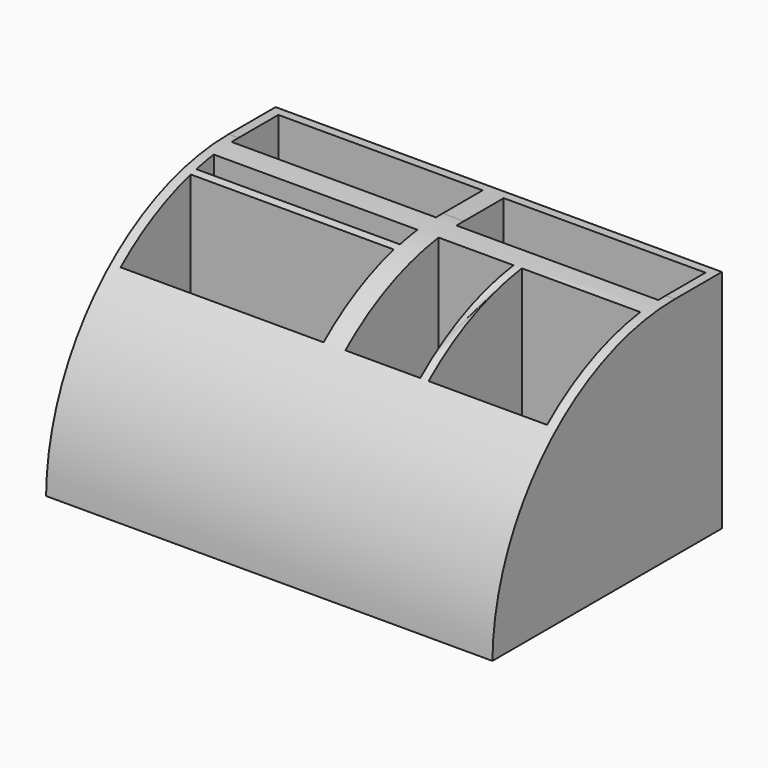
from build123d import *

# Parameters (mm, degrees)
F0_W        = 198.8127231598
F0_H        = 127.7878135443
F1_DEPTH    = 100.584
F2_T1_DEPTH = 706.7873225248
F3_W        = 90.9917657264
F3_H        = 25.9568989277
F4_DEPTH    = 88.392
F5_W        = 89.8508075625
F5_H        = 26.2421388179
F6_DEPTH    = 88.646
F7_DEPTH    = 0.254
F8_DEPTH    = 0.254
F9_W        = 90.7065253705
F9_H        = 9.6981823444
F10_DEPTH   = 90.678
F11_W       = 90.4212845489
F11_H       = 39.0779660083
F11_W_2     = 33.3731551655
F11_H_2     = 51.9137959927
F11_W_3     = 52.7695268393
F12_DEPTH   = 88.646


# Not quite as in the source:
# - a fillet or chamfer that OpenCascade refuses, or shapes differently, is made with other operations: its cross-section is extruded or revolved along the edge and cut away or added


with BuildPart() as f1:
    # F0 (on Top) → F1 (new body)
    with BuildSketch(Plane.XY):
        with Locations((-0.7131025195, -5.5621936917)):
            Rectangle(F0_W, F0_H)
    extrude(amount=-F1_DEPTH)

    # F2: fillet of radius 101.6 on 1 edges, made by hand

    # F2_s2 → F2_t1 (cut)
    with BuildSketch(Plane.YZ.offset(-354.1067637819)):
        with BuildLine():
            ThreePointArc((-69.4561004639, -100.584), (-39.3431167706, -29.39963435), (32.1388194091, 0))
            Line((32.1388194091, 0), (-69.4561004639, 0))
            Line((-69.4561004639, 0), (-69.4561004639, -100.584))
        make_face()
    extrude(amount=F2_T1_DEPTH, mode=Mode.SUBTRACT)

    # F3 (on Top) → F4 (cut)
    with BuildSketch(Plane.XY):
        with Locations((-50.2023545559, 41.3598939776)):
            Rectangle(F3_W, F3_H)
    extrude(amount=-F4_DEPTH, mode=Mode.SUBTRACT)

    # F5 (on Top) → F6 (cut)
    with BuildSketch(Plane.XY):
        with Locations((49.631874077, 41.2172740325)):
            Rectangle(F5_W, F5_H)
    extrude(amount=-F6_DEPTH, mode=Mode.SUBTRACT)

    # F7 (cut): a face of the model
    f7_faces = [f1.faces().sort_by_distance(p)[0] for p in [
        (-50.2023545559, 41.3598939776, -88.392),
    ]]
    extrude(f7_faces, amount=F7_DEPTH, mode=Mode.SUBTRACT)

    # F8 (cut): a face of the model
    f8_faces = [f1.faces().sort_by_distance(p)[0] for p in [
        (49.631874077, 41.2172740325, -88.646),
    ]]
    extrude(f8_faces, amount=-F8_DEPTH, mode=Mode.SUBTRACT)

    # F9 (on Top) → F10 (cut)
    with BuildSketch(Plane.XY):
        with Locations((-50.3449747339, 13.5489311069)):
            Rectangle(F9_W, F9_H)
    extrude(amount=-F10_DEPTH, mode=Mode.SUBTRACT)

    # F11 (on Top) → F12 (cut)
    with BuildSketch(Plane.XY):
        with Locations((-50.4875951447, -13.9767907094)):
            Rectangle(F11_W, F11_H)
        with Locations((21.1078075226, -7.5588757172)):
            Rectangle(F11_W_2, F11_H_2)
        with Locations((67.8872764111, -7.5588757172)):
            Rectangle(F11_W_3, F11_H_2)
    extrude(amount=-F12_DEPTH, mode=Mode.SUBTRACT)


solid = f1.part
